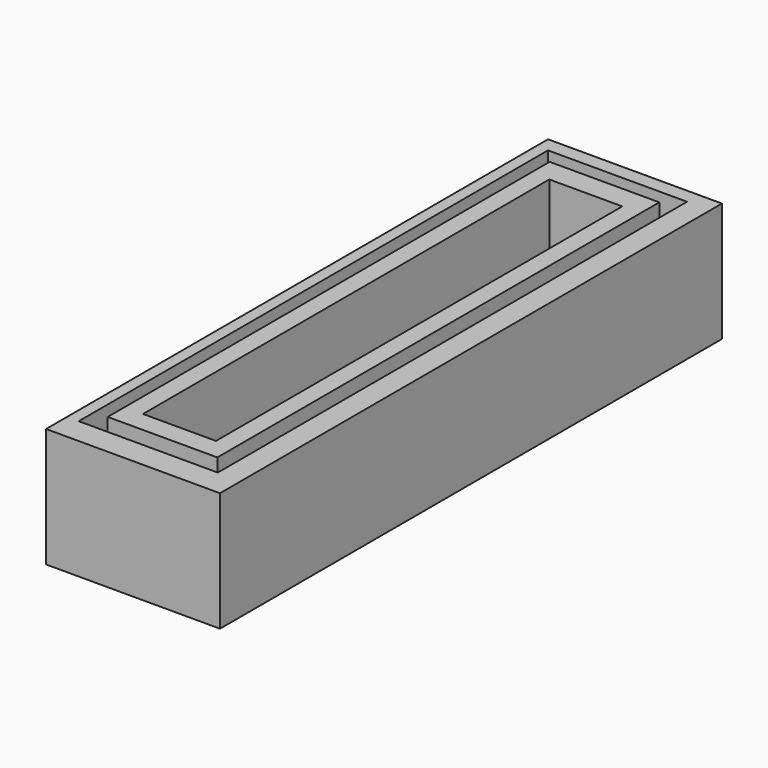
from build123d import *

# Parameters (mm, degrees)
F0_W     = 324.6865719557
F0_H     = 61.7302879691
F1_DEPTH = 90
F3_W     = 71.9730192795
F3_H     = 303.5411946476
F3_W_2   = 56.7419305444
F3_H_2   = 285.8860269189
F3_W_3   = 37.7663187683
F3_H_3   = 262.8358900547
F4_DEPTH = 61.7312879691


# Not quite as in the source:
# - the program builds the solid bodies; features that only make, move or delete a surface that nothing else refers to are left out


with BuildPart() as f1:
    # F0 (on Right) → F1 (new body)
    with BuildSketch(Plane.YZ):
        with Locations((-198.1138437986, 64.6366849542)):
            Rectangle(F0_W, F0_H)
    extrude(amount=F1_DEPTH)

    # F3 (on face) → F4 (cut, through all)
    with BuildSketch(Plane.XY.offset(95.5018289387)):
        with Locations((42.0340183191, -195.1250378042)):
            Rectangle(F3_W, F3_H)
        with Locations((41.2159748375, -193.7081329525)):
            Rectangle(F3_W_2, F3_H_2, mode=Mode.SUBTRACT)
        with Locations((41.2525031716, -194.3167597055)):
            Rectangle(F3_W_3, F3_H_3)
    extrude(amount=-F4_DEPTH, mode=Mode.SUBTRACT)


solid = f1.part
